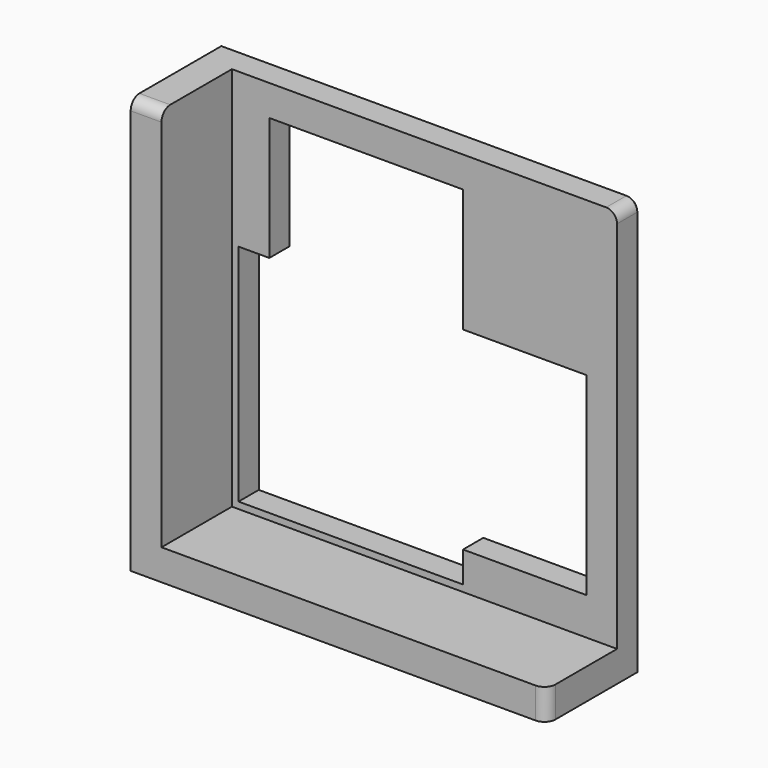
from build123d import *

# Parameters (mm, degrees)
F0_W        = 7
F0_H        = 7
F0_W_2      = 35
F0_H_2      = 52.5
F0_H_3      = 35
F1_DEPTH    = 20
F0_W_3      = 51
F0_H_4      = 1.5
F2_DEPTH    = 7
F3_T1_DEPTH = 19.49950001
F3_T3_DEPTH = 19.49950001
F3_T5_DEPTH = 19.49950001
F4_SIZE     = 1.25


# Not quite as in the source:
# - a fillet or chamfer that OpenCascade refuses, or shapes differently, is made with other operations: its cross-section is extruded or revolved along the edge and cut away or added


with BuildPart() as f1:
    # F0 (on Front) → F1 (new body)
    with BuildSketch(Plane.XZ):
        with Locations((-26.1161934872, -30.8009498573)):
            Rectangle(F0_W, F0_H)
        with Locations((47.3838065128, -30.8009498573)):
            Rectangle(F0_W_2, F0_H)
        with Locations((-26.1161934872, -1.0509498573)):
            Rectangle(F0_W, F0_H_2)
        Polygon((-21.1161934872, -27.3009498573), (-22.6161934872, -27.3009498573), (-22.6161934872, -34.3009498573), (29.8838065128, -34.3009498573), (29.8838065128, -27.3009498573), align=None)
        with Locations((-26.1161934872, 42.6990501427)):
            Rectangle(F0_W, F0_H_3)
    extrude(amount=F1_DEPTH)

    # F0 (on Front) + F1_face (on face) → F2 (join)
    with BuildSketch(Plane.XZ):
        Polygon((-22.6161934872, 60.1990501427), (-22.6161934872, 25.1990501427), (-21.1161934872, 25.1990501427), (-14.1161934872, 25.1990501427), (-14.1161934872, 53.1990501427), (29.8838065128, 53.1990501427), (29.8838065128, 60.1990501427), align=None)
        Polygon((-21.1161934872, -27.3009498573), (-22.6161934872, -27.3009498573), (-22.6161934872, -34.3009498573), (29.8838065128, -34.3009498573), (29.8838065128, -27.3009498573), align=None)
        with Locations((-26.1161934872, 42.6990501427)):
            Rectangle(F0_W, F0_H_3)
        with Locations((-26.1161934872, -1.0509498573)):
            Rectangle(F0_W, F0_H_2)
        Polygon((29.8838065128, -18.8009498573), (29.8838065128, -25.8009498573), (29.8838065128, -27.3009498573), (64.8838065128, -27.3009498573), (64.8838065128, 25.1990501427), (57.8838065128, 25.1990501427), (57.8838065128, -18.8009498573), align=None)
        with Locations((-26.1161934872, -30.8009498573)):
            Rectangle(F0_W, F0_H)
        Polygon((64.8838065128, 60.1990501427), (29.8838065128, 60.1990501427), (29.8838065128, 53.1990501427), (29.8838065128, 25.1990501427), (57.8838065128, 25.1990501427), (64.8838065128, 25.1990501427), align=None)
        with Locations((47.3838065128, -30.8009498573)):
            Rectangle(F0_W_2, F0_H)
        Polygon((-21.1161934872, 25.1990501427), (-22.6161934872, 25.1990501427), (-22.6161934872, -27.3009498573), (-21.1161934872, -27.3009498573), (-21.1161934872, -25.8009498573), align=None)
        with Locations((4.3838065128, -26.5509498573)):
            Rectangle(F0_W_3, F0_H_4)
    with BuildSketch(Plane(origin=(-3.3998473333, -20, -8.0846037034), x_dir=(1, 0, 0), z_dir=(0, -1, 0))):
        Polygon((-26.2163461538, -26.2163461538), (68.2836538462, -26.2163461538), (68.2836538462, -19.2163461538), (-19.2163461538, -19.2163461538), (-19.2163461538, 68.2836538462), (-26.2163461538, 68.2836538462), align=None)
    extrude(amount=F2_DEPTH)

    # F3: fillet of radius 2.5 on 3 edges, made by hand

    # F3_s2 → F3_t1 (cut)
    with BuildSketch(Plane.YZ.offset(-35.8659434922)):
        with BuildLine():
            ThreePointArc((-24.5001, 60.1991501427), (-26.267866953, 59.4669170957), (-27.0001, 57.6991501427))
            Line((-27.0001, 57.6991501427), (-27.0501, 57.6991501427))
            ThreePointArc((-27.0501, 57.6991501427), (-27.05, 58.9491001427), (-27.05, 60.1990501427))
            Line((-27.05, 60.1990501427), (-27, 60.2490501427))
            ThreePointArc((-27, 60.2490501427), (-25.75005, 60.2490501427), (-24.5001, 60.2491501427))
            Line((-24.5001, 60.2491501427), (-24.5001, 60.1991501427))
        make_face()
    extrude(amount=F3_T1_DEPTH, mode=Mode.SUBTRACT)

    # F3_s4 → F3_t3 (cut)
    with BuildSketch(Plane.XY.offset(-40.5506998623)):
        with BuildLine():
            ThreePointArc((64.8839065128, -24.5001), (64.1516734658, -26.267866953), (62.3839065128, -27.0001))
            Line((62.3839065128, -27.0001), (62.3839065128, -27.0501))
            ThreePointArc((62.3839065128, -27.0501), (63.6338565128, -27.05), (64.8838065128, -27.05))
            Line((64.8838065128, -27.05), (64.9338065128, -27))
            ThreePointArc((64.9338065128, -27), (64.9338065128, -25.75005), (64.9339065128, -24.5001))
            Line((64.9339065128, -24.5001), (64.8839065128, -24.5001))
        make_face()
    extrude(amount=F3_T3_DEPTH, mode=Mode.SUBTRACT)

    # F3_s6 → F3_t5 (cut)
    with BuildSketch(Plane.XZ.offset(-6.249750005)):
        with BuildLine():
            ThreePointArc((64.8839065128, 57.6991501427), (64.1516734658, 59.4669170957), (62.3839065128, 60.1991501427))
            Line((62.3839065128, 60.1991501427), (62.3839065128, 60.2491501427))
            ThreePointArc((62.3839065128, 60.2491501427), (63.6338565128, 60.2490501427), (64.8838065128, 60.2490501427))
            Line((64.8838065128, 60.2490501427), (64.9338065128, 60.1990501427))
            ThreePointArc((64.9338065128, 60.1990501427), (64.9338065128, 58.9491001427), (64.9339065128, 57.6991501427))
            Line((64.9339065128, 57.6991501427), (64.8839065128, 57.6991501427))
        make_face()
    extrude(amount=F3_T5_DEPTH, mode=Mode.SUBTRACT)

    # F4
    f4_edges = [f1.edges().sort_by_distance(p)[0] for p in [
        (43.883807, 0, 25.19905),
        (57.883807, 0, 3.19905),
        (43.883807, 0, -18.80095),
        (29.883807, 0, -22.30095),
        (4.383807, 0, -25.80095),
        (-21.116193, 0, -0.30095),
        (29.883807, 0, 39.19905),
        (7.883807, 0, 53.19905),
        (-14.116193, 0, 39.19905),
        (-17.616193, 0, 25.19905),
        (64.883807, 0, 11.71028),
        (16.395037, 0, 60.19905),
        (64.151673, 0, 59.466917),
    ]]
    chamfer(f4_edges, length=F4_SIZE)


solid = f1.part
